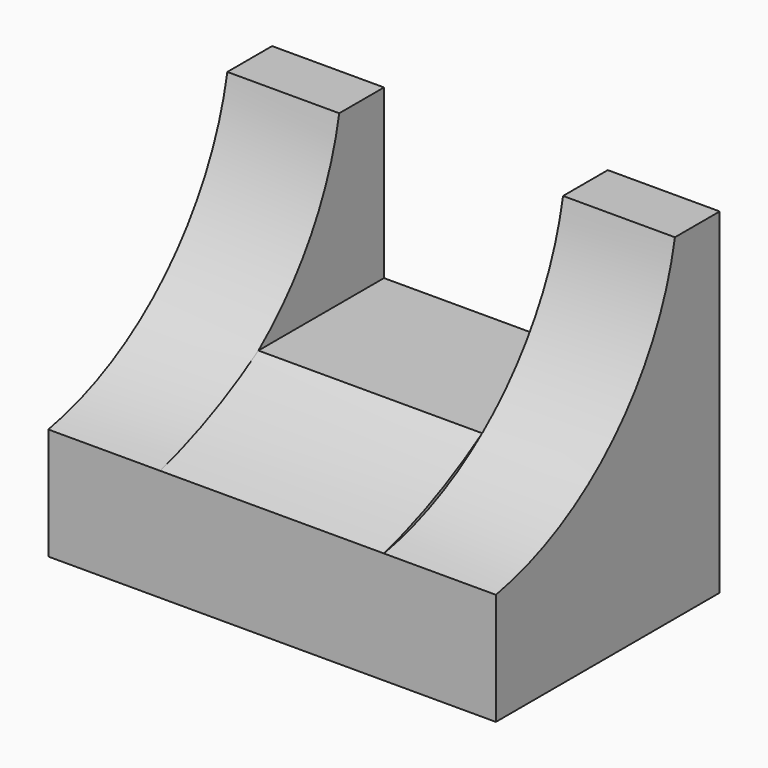
from build123d import *

# Parameters (mm, degrees)
F0_W     = 50.8
F0_H     = 38.1
F1_DEPTH = 31.75
F2_W     = 25.4
F2_H     = 19.05
F3_DEPTH = 31.75
F5_DEPTH = 12.7
F7_DEPTH = 12.7
F9_DEPTH = 25.4


with BuildPart() as f1:
    # F0 (on Front) → F1 (new body)
    with BuildSketch(Plane.XZ):
        with Locations((25.4, 19.05)):
            Rectangle(F0_W, F0_H)
    extrude(amount=F1_DEPTH)

    # F2 (on face) → F3 (cut)
    with BuildSketch(Plane.XZ.offset(31.75)):
        with Locations((25.4, 28.575)):
            Rectangle(F2_W, F2_H)
    extrude(amount=-F3_DEPTH, mode=Mode.SUBTRACT)

    # F4 (on face) → F5 (cut)
    with BuildSketch(Plane.YZ.offset(50.8)):
        with BuildLine():
            Line((-31.75, 38.1), (-31.75, 12.7))
            ThreePointArc((-31.75, 12.7), (-15.1126319635, 21.4626319635), (-6.35, 38.1))
            Line((-6.35, 38.1), (-31.75, 38.1))
        make_face()
    extrude(amount=-F5_DEPTH, mode=Mode.SUBTRACT)

    # F6 (on face) → F7 (cut)
    with BuildSketch(Plane(origin=(0, 0, 0), x_dir=(0, -1, 0), z_dir=(-1, 0, 0))):
        with BuildLine():
            Line((31.75, 38.1), (6.35, 38.1))
            ThreePointArc((6.35, 38.1), (15.1126319635, 21.4626319635), (31.75, 12.7))
            Line((31.75, 12.7), (31.75, 38.1))
        make_face()
    extrude(amount=-F7_DEPTH, mode=Mode.SUBTRACT)

    # F8 (on face) → F9 (cut)
    with BuildSketch(Plane.YZ.offset(38.1)):
        with BuildLine():
            Line((-31.75, 19.05), (-31.75, 12.7))
            ThreePointArc((-31.75, 12.7), (-24.5433360644, 15.3470979527), (-17.8178881924, 19.05))
            Line((-17.8178881924, 19.05), (-31.75, 19.05))
        make_face()
    extrude(amount=-F9_DEPTH, mode=Mode.SUBTRACT)


solid = f1.part
